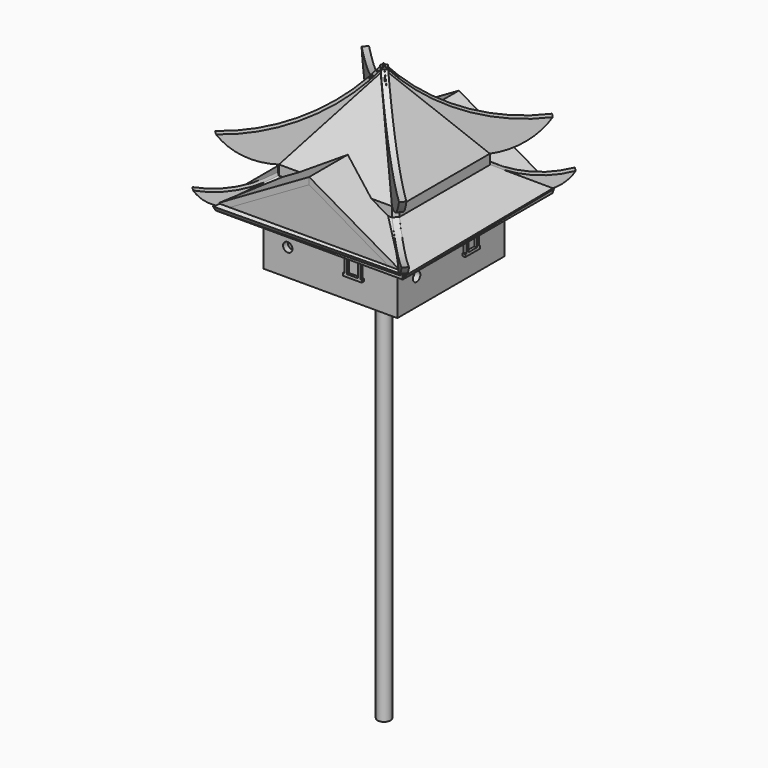
from build123d import *

# Parameters (mm, degrees)
F0_R             = 24.15
F0_R_2           = 21.55
F1_DEPTH         = 1500
F5_COUNT         = 4
F6_W             = 500
F6_H             = 500
F7_DEPTH         = 200
F8_T             = -22
F10_DEPTH        = 178
F11_R            = 17.5
F12_DEPTH        = 25
F12_COPIES_COUNT = 4
F13_W            = 700
F13_H            = 700
F14_DEPTH        = 22
F15_W            = 10
F15_H            = 60
F16_DEPTH        = 10
F17_COUNT        = 4
F19_DEPTH        = 700
F22_DEPTH        = 22
F28_DEPTH        = 11
F29_COUNT        = 4
F31_W            = 423.2943853771
F31_H            = 36.439377683
F32_DEPTH        = 22
F36_DEPTH        = 22
F39_DEPTH        = 22
F40_COUNT        = 4


# Not quite as in the source:
# - a pattern or mirror of a feature is missing from the dataset's text; its kind, count and spacing are read off the source's solid


with BuildPart() as f1:
    # F0 (on Top) → F1 (new body)
    with BuildSketch(Plane.XY):
        with Locations((0, -200)):
            Circle(F0_R)
        with Locations((0, -200)):
            Circle(F0_R_2, mode=Mode.SUBTRACT)
    extrude(amount=F1_DEPTH)


with BuildPart() as f4:
    # F3 (on offset) → F4 (new body, up to the next surface of F1)
    with BuildSketch(Plane.XZ.offset(85)):
        Polygon((13.6246460956, 1500), (-11.3753539044, 1500), (-11.3753539044, 1475), (-8.3753539044, 1475), (-8.3753539044, 1497), (13.6246460956, 1497), align=None)
    extrude(until=Until.NEXT, target=f1.part)


with BuildPart() as f5_1:
    # F5: instance of F4
    add(f4.part.rotate(Axis((0, -200, 1500), (0, 0, 1)), 1 * 360 / F5_COUNT))


with BuildPart() as f5_2:
    # F5: instance of F4
    add(f4.part.rotate(Axis((0, -200, 1500), (0, 0, 1)), 2 * 360 / F5_COUNT))


with BuildPart() as f5_3:
    # F5: instance of F4
    add(f4.part.rotate(Axis((0, -200, 1500), (0, 0, 1)), 3 * 360 / F5_COUNT))


with BuildPart() as f7:
    # F6 (on face) → F7 (new body)
    with BuildSketch(Plane.XY.offset(1500)):
        with Locations((0, -200)):
            Rectangle(F6_W, F6_H)
    extrude(amount=F7_DEPTH)

    # F8
    f8_openings = [f7.faces().sort_by_distance(p)[0] for p in [
        (0, -200, 1700),
    ]]
    offset(amount=F8_T, openings=f8_openings)

    # F11 (on face) → F12 (cut)
    with BuildSketch(Plane.YZ.offset(250)):
        with Locations((-360, 1600)):
            Circle(F11_R)
    f12 = extrude(amount=-F12_DEPTH, mode=Mode.SUBTRACT)

    # F12_copies: F12 ×4 about axis
    f12_copies_axis = Axis((0, -200, 0), (0, 0, 1))
    for i in range(1, F12_COPIES_COUNT):
        add(f12.rotate(f12_copies_axis, i * 360 / F12_COPIES_COUNT), mode=Mode.SUBTRACT)


with BuildPart() as f10:
    # F9 (on face) → F10 (new body, through all)
    with BuildSketch(Plane.XY.offset(1522)):
        Polygon((228, -211), (228, -189), (11, -189), (11, 28), (-11, 28), (-11, -189), (-228, -189), (-228, -211), (-11, -211), (-11, -428), (11, -428), (11, -211), align=None)
    extrude(amount=F10_DEPTH)


with BuildPart() as f14:
    # F13 (on face) → F14 (new body)
    with BuildSketch(Plane.XY.offset(1700)):
        with Locations((0, -200)):
            Rectangle(F13_W, F13_H)
    extrude(amount=F14_DEPTH)


with BuildPart() as f16:
    # F15 (on face) → F16 (new body)
    with BuildSketch(Plane.XZ.offset(450)):
        Polygon((55, 1650), (60, 1650), (70, 1650), (110, 1650), (120, 1650), (125, 1650), (125, 1660), (55, 1660), align=None)
        with Locations((65, 1620)):
            Rectangle(F15_W, F15_H)
        Polygon((70, 1590), (60, 1590), (55, 1590), (55, 1580), (125, 1580), (125, 1590), (120, 1590), (110, 1590), align=None)
        with Locations((115, 1620)):
            Rectangle(F15_W, F15_H)
    extrude(amount=F16_DEPTH)


with BuildPart() as f17_1:
    # F17: instance of F16
    add(f16.part.rotate(Axis((0, -200, 0), (0, 0, 1)), 1 * 360 / F17_COUNT))


with BuildPart() as f17_2:
    # F17: instance of F16
    add(f16.part.rotate(Axis((0, -200, 0), (0, 0, 1)), 2 * 360 / F17_COUNT))


with BuildPart() as f17_3:
    # F17: instance of F16
    add(f16.part.rotate(Axis((0, -200, 0), (0, 0, 1)), 3 * 360 / F17_COUNT))


with BuildPart() as f19:
    # F18 (on face) → F19 (new body, through all)
    with BuildSketch(Plane.XZ.offset(550)):
        Polygon((0, 1898.669182372), (0, 1924.0725942164), (-350, 1722), (-306, 1722), align=None)
    extrude(amount=-F19_DEPTH)


with BuildPart() as f20_1:
    # F20: instance of F19
    add(f19.part.mirror(Plane.YZ))


with BuildPart() as f22:
    # F21 (on face) → F22 (new body)
    with BuildSketch(Plane.XZ.offset(550)):
        Polygon((0, 1898.669182372), (-306, 1722), (306, 1722), align=None)
    extrude(amount=-F22_DEPTH)


with BuildPart() as f24_1:
    # F24: instance of F22
    add(f22.part.mirror(Plane(origin=(0, -200, 1600), x_dir=(1, 0, 0), z_dir=(0, -1, 0))))


with BuildPart() as f28:
    # F27 (on face) → F28 (new body, symmetric)
    with BuildSketch(Plane(origin=(100, -100, 0), x_dir=(-0.7071067812, -0.7071067812, 0), z_dir=(-0.7071067812, 0.7071067812, 0))):
        with BuildLine():
            ThreePointArc((636.3961030679, 1956.2034019503), (365.9890865624, 1996.2714682153), (141.4213562373, 2152.1391653377))
            Line((141.4213562373, 2152.1391653377), (141.4213562373, 1722))
            Line((141.4213562373, 1722), (636.3961030679, 1722))
            ThreePointArc((636.3961030679, 1722), (674.6845307285, 1742.6983610818), (703.5547499331, 1775.2703780179))
            ThreePointArc((703.5547499331, 1775.2703780179), (574.579078085, 1769.1105431654), (452.1469186165, 1810.1353383745))
            Line((452.1469186165, 1810.1353383745), (451.3244545349, 1846.5700748542))
            ThreePointArc((451.3244545349, 1846.5700748542), (556.2545348635, 1880.464036679), (636.3961030679, 1956.2034019503))
        make_face()
    extrude(amount=F28_DEPTH, both=True)


with BuildPart() as f29_1:
    # F29: instance of F28
    add(f28.part.rotate(Axis((0, -200, 0), (0, 0, 1)), 1 * 360 / F29_COUNT))


with BuildPart() as f29_2:
    # F29: instance of F28
    add(f28.part.rotate(Axis((0, -200, 0), (0, 0, 1)), 2 * 360 / F29_COUNT))


with BuildPart() as f29_3:
    # F29: instance of F28
    add(f28.part.rotate(Axis((0, -200, 0), (0, 0, 1)), 3 * 360 / F29_COUNT))


with BuildPart() as f32:
    # F31 (on 3pt) → F32 (new body)
    with BuildSketch(Plane(origin=(0, -456.271390046, 7.2829872187), x_dir=(-1, 0, 0), z_dir=(0, 0.9998726322, -0.0159599303))):
        with Locations((-0.2907849647, 1821.3016945847)):
            Rectangle(F31_W, F31_H)
    extrude(amount=F32_DEPTH)


with BuildPart() as f36:
    # F35 (on 3pt) → F36 (new body)
    with BuildSketch(Plane(origin=(0, -1159.0247896943, 860.6809999676), x_dir=(-1, 0, 0), z_dir=(0, 0.802846245, -0.5961861344))):
        Polygon((211.3564077239, 1227.9923845564), (0, 1608.5996208346), (-211.3564077239, 1227.9923845564), align=None)
    extrude(amount=F36_DEPTH)


with BuildPart() as f39:
    # F38 (on 3pt) → F39 (new body)
    with BuildSketch(Plane(origin=(0, -974.2971667202, 1440.2302876105), x_dir=(1, 0, 0), z_dir=(0, -0.560318733, 0.8282770777))):
        Polygon((211.9379776533, 660.1689876709), (-211.9379776533, 660.1689876709), (-350, 496.9894534457), (342.2218254069, 502.873981851), align=None)
    extrude(amount=-F39_DEPTH)


with BuildPart() as f40_1:
    # F40: instance of F39
    add(f39.part.rotate(Axis((0, -200, 0), (0, 0, 1)), 1 * 360 / F40_COUNT))


with BuildPart() as f40_2:
    # F40: instance of F39
    add(f39.part.rotate(Axis((0, -200, 0), (0, 0, 1)), 2 * 360 / F40_COUNT))


with BuildPart() as f40_3:
    # F40: instance of F39
    add(f39.part.rotate(Axis((0, -200, 0), (0, 0, 1)), 3 * 360 / F40_COUNT))


with BuildPart() as f40_4:
    # F40: instance of F32
    add(f32.part.rotate(Axis((0, -200, 0), (0, 0, 1)), 1 * 360 / F40_COUNT))


with BuildPart() as f40_5:
    # F40: instance of F32
    add(f32.part.rotate(Axis((0, -200, 0), (0, 0, 1)), 2 * 360 / F40_COUNT))


with BuildPart() as f40_6:
    # F40: instance of F32
    add(f32.part.rotate(Axis((0, -200, 0), (0, 0, 1)), 3 * 360 / F40_COUNT))


with BuildPart() as f40_7:
    # F40: instance of F36
    add(f36.part.rotate(Axis((0, -200, 0), (0, 0, 1)), 1 * 360 / F40_COUNT))


with BuildPart() as f40_8:
    # F40: instance of F36
    add(f36.part.rotate(Axis((0, -200, 0), (0, 0, 1)), 2 * 360 / F40_COUNT))


with BuildPart() as f40_9:
    # F40: instance of F36
    add(f36.part.rotate(Axis((0, -200, 0), (0, 0, 1)), 3 * 360 / F40_COUNT))


solid = Compound([f1.part, f4.part, f5_1.part, f5_2.part, f5_3.part, f7.part, f10.part, f14.part, f16.part, f17_1.part, f17_2.part, f17_3.part, f19.part, f20_1.part, f22.part, f24_1.part, f28.part, f29_1.part, f29_2.part, f29_3.part, f32.part, f36.part, f39.part, f40_1.part, f40_2.part, f40_3.part, f40_4.part, f40_5.part, f40_6.part, f40_7.part, f40_8.part, f40_9.part])
